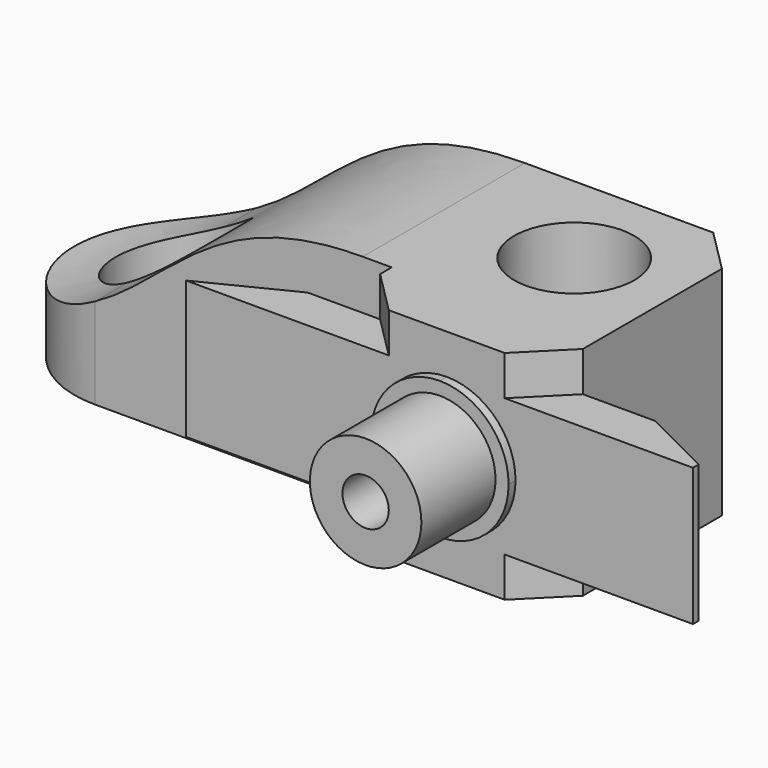
from build123d import *

# Parameters (mm, degrees)
F0_R         = 4.15
F1_DEPTH     = 15
F2_W         = 14
F2_H         = 15
F3_DEPTH     = 4
F4_R         = 3.85
F5_DEPTH     = 3
F6_T1_DEPTH  = 40.5779464854
F4_R_2       = 1.6
F7_DEPTH     = 7
F8_DEPTH     = 0.6
F10_DEPTH    = 25
F11_T1_DEPTH = 30.4300979278
F11_T3_DEPTH = 10.4650489639
F11_T5_DEPTH = 10.4650489639


# Not quite as in the source:
# - a fillet or chamfer that OpenCascade refuses, or shapes differently, is made with other operations: its cross-section is extruded or revolved along the edge and cut away or added


with BuildPart() as f1:
    # F0 (on Top) → F1 (new body)
    with BuildSketch(Plane.XY):
        with BuildLine():
            Line((7, 7), (-27.5, 7))
            ThreePointArc((-27.5, 7), (-34.5, 0), (-27.5, -7))
            Line((-27.5, -7), (7, -7))
            Line((7, -7), (7, 7))
        make_face()
        with Locations((-27.5, 0)):
            Circle(F0_R, mode=Mode.SUBTRACT)
        Circle(F0_R, mode=Mode.SUBTRACT)
    extrude(amount=F1_DEPTH)

    # F2 (on face) → F3 (join)
    with BuildSketch(Plane.XZ.offset(7)):
        with Locations((0, 7.5)):
            Rectangle(F2_W, F2_H)
    extrude(amount=F3_DEPTH)

    # F4 (on face) → F5 (join)
    with BuildSketch(Plane.XZ.offset(11)):
        with BuildLine():
            ThreePointArc((0, 2.75), (3.3587572106, 4.1412427894), (4.75, 7.5))
            ThreePointArc((4.75, 7.5), (3.3587572106, 10.8587572106), (0, 12.25))
            ThreePointArc((0, 12.25), (-4.75, 7.5), (0, 2.75))
        make_face()
        with Locations((0, 7.5)):
            Circle(F4_R, mode=Mode.SUBTRACT)
        with BuildLine():
            ThreePointArc((0, 12.25), (3.3587572106, 10.8587572106), (4.75, 7.5))
            ThreePointArc((4.75, 7.5), (3.3587572106, 4.1412427894), (0, 2.75))
            Line((0, 2.75), (18, 2.75))
            Line((18, 2.75), (18, 12.25))
            Line((18, 12.25), (0, 12.25))
        make_face()
        with BuildLine():
            ThreePointArc((0, 2.75), (-4.75, 7.5), (0, 12.25))
            Line((0, 12.25), (-18, 12.25))
            Line((-18, 12.25), (-18, 2.75))
            Line((-18, 2.75), (0, 2.75))
        make_face()
    extrude(amount=-F5_DEPTH)

    # F6: chamfer of 3 x 6 on 2 edges, made by hand

    # F6_s2 → F6_t1 (cut)
    with BuildSketch(Plane.XY.offset(-12.7889732427)):
        Polygon((-12, -8), (-18, -11), (-18, -8), align=None)
        Polygon((12, -8), (18, -11), (18, -8), align=None)
    extrude(amount=F6_T1_DEPTH, mode=Mode.SUBTRACT)

    # F4 (on face) → F7 (join)
    with BuildSketch(Plane.XZ.offset(11)):
        with Locations((0, 7.5)):
            Circle(F4_R)
        with Locations((0, 7.5)):
            Circle(F4_R_2, mode=Mode.SUBTRACT)
    extrude(amount=F7_DEPTH)

    # F4 (on face) → F8 (join)
    with BuildSketch(Plane.XZ.offset(11)):
        with BuildLine():
            ThreePointArc((0, 2.75), (3.3587572106, 4.1412427894), (4.75, 7.5))
            ThreePointArc((4.75, 7.5), (3.3587572106, 10.8587572106), (0, 12.25))
            ThreePointArc((0, 12.25), (-4.75, 7.5), (0, 2.75))
        make_face()
        with Locations((0, 7.5)):
            Circle(F4_R, mode=Mode.SUBTRACT)
    extrude(amount=F8_DEPTH)

    # F9 (on face) → F10 (intersect, symmetric)
    with BuildSketch(Plane.XZ.offset(7)):
        with BuildLine():
            Line((-27.5, 6.2586253838), (-27.5, 0))
            Line((-27.5, 0), (-7, 0))
            Line((-7, 0), (-7, 15))
            Line((-7, 15), (-9, 15))
            add(Edge.make_bspline(
                [(-27.5, 6.2586253838), (-22.0570868036, 9.2486118384), (-19.3657420182, 15), (-9, 15)],
                knots=[7.0475438496, 7.0475438496, 7.0475438496, 7.0475438496, 27.5771644663, 27.5771644663, 27.5771644663, 27.5771644663], degree=3))
        make_face()
        with BuildLine():
            Line((-34.5, 4.5), (-34.5, 0))
            Line((-34.5, 0), (-27.5, 0))
            Line((-27.5, 0), (-27.5, 6.2586253838))
            add(Edge.make_bspline(
                [(-34.5, 4.5), (-31.5612189253, 4.5312000669), (-29.3684792153, 5.2322030722), (-27.5, 6.2586253838)],
                knots=[0, 0, 0, 0, 7.0475438496, 7.0475438496, 7.0475438496, 7.0475438496], degree=3))
        make_face()
        Polygon((-7, 15), (-7, 0), (0, 0), (17, 0), (17, 15), align=None)
    extrude(amount=F10_DEPTH, both=True, mode=Mode.INTERSECT)

    # F11: chamfer of 3 on 6 edges, made by hand

    # F11_s2 → F11_t1 (cut)
    with BuildSketch(Plane.XY.offset(-7.7150489639)):
        Polygon((4, 7), (7, 4), (7, 7), align=None)
    extrude(amount=F11_T1_DEPTH, mode=Mode.SUBTRACT)

    # F11_s4 → F11_t3 (cut)
    with BuildSketch(Plane.XY.offset(12.25)):
        Polygon((-4, -11), (-7, -8), (-7, -11), align=None)
        Polygon((7, -8), (4, -11), (7, -11), align=None)
    extrude(amount=F11_T3_DEPTH, mode=Mode.SUBTRACT)

    # F11_s6 → F11_t5 (cut)
    with BuildSketch(Plane.XY.offset(-7.7150489639)):
        Polygon((-4, -11), (-7, -8), (-7, -11), align=None)
        Polygon((7, -8), (4, -11), (7, -11), align=None)
    extrude(amount=F11_T5_DEPTH, mode=Mode.SUBTRACT)


solid = f1.part
